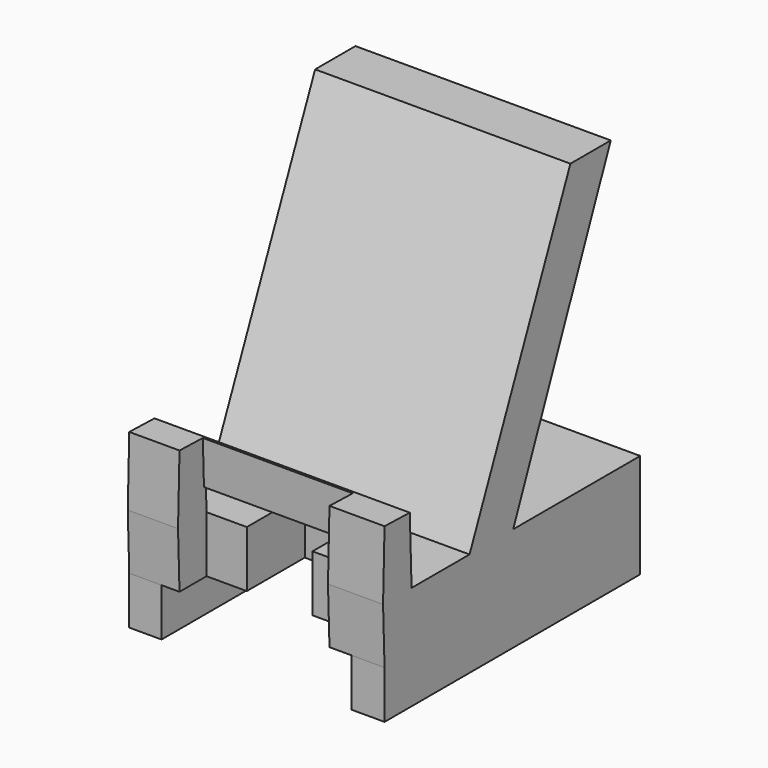
from build123d import *

# Parameters (mm, degrees)
F1_DEPTH  = 80
F2_W      = 10.1163312793
F2_H      = 100.1585014164
F2_W_2    = 10.3900524974
F3_DEPTH  = 15
F6_W      = 19.9106484652
F6_H      = 22.7042857278
F7_DEPTH  = 17.6
F8_W      = 20.5874107778
F8_H      = 22.7042857278
F9_DEPTH  = 17.7
F10_W     = 46.9934158027
F10_H     = 17.6760927897
F10_H_2   = 21.9856097649
F11_DEPTH = 10.4
F13_DEPTH = 25
F15_DEPTH = 25


# Not quite as in the source:
# - a feature of the source that left no trace in its solid (it failed there, or was rolled back) is left out


with BuildPart() as f1:
    # F0 (on Right) → F1 (new body)
    with BuildSketch(Plane.YZ):
        Polygon((22.4307589233, 109.4066873193), (-17.082426697, 17.6664423198), (0, 17.6664423198), (38.2366999984, 109.4066873193), align=None)
        Polygon((-39.7867124248, 17.6664423198), (-39.2026986647, 0), (49.7872419655, 0), (49.7872419655, 17.6664423198), (0, 17.6664423198), (-17.082426697, 17.6664423198), align=None)
        Polygon((-50.955273211, 17.6664423198), (-50.3712594509, 0), (-39.2026986647, 0), (-39.7867124248, 17.6664423198), align=None)
        Polygon((-50.3712594509, 38.982976228), (-50.955273211, 17.6664423198), (-39.7867124248, 17.6664423198), (-40.4824339626, 38.7120499047), align=None)
    extrude(amount=F1_DEPTH)

    # F2 (on face) → F3 (join)
    with BuildSketch(Plane(origin=(0, 0, 0), x_dir=(1, 0, 0), z_dir=(0, 0, -1))):
        with Locations((5.0581656396, 0.2920087427)):
            Rectangle(F2_W, F2_H)
        with Locations((74.8049737513, 0.2920087427)):
            Rectangle(F2_W_2, F2_H)
    extrude(amount=F3_DEPTH)

    # F6 (on face) → F7 (join)
    with BuildSketch(Plane.XY.offset(17.6664423198)):
        with Locations((39.5665168762, -28.4345695609)):
            Rectangle(F6_W, F6_H)
    extrude(amount=-F7_DEPTH)

    # F8 (on face) → F9 (cut)
    with BuildSketch(Plane.XY.offset(17.6664423198)):
        with Locations((38.6653598398, -28.4345695609)):
            Rectangle(F8_W, F8_H)
    extrude(amount=-F9_DEPTH, mode=Mode.SUBTRACT)

    # F10 (on face) → F11 (cut)
    with BuildSketch(Plane(origin=(0, -50.316272907, -1.6633454095), x_dir=(1, 0, 0), z_dir=(0, -0.9994540383, -0.0330397541))):
        with Locations((39.2467323691, 10.5023004233)):
            Rectangle(F10_W, F10_H)
        with Locations((39.2467323691, 30.3331517006)):
            Rectangle(F10_W, F10_H_2)
    extrude(amount=-F11_DEPTH, mode=Mode.SUBTRACT)

    # F12 (on face) → F13 (cut)
    with BuildSketch(Plane(origin=(0, 0, 0), x_dir=(1, 0, 0), z_dir=(0, 0, -1))):
        Polygon((62.7434402704, 50.3712594509), (15.7500244677, 50.3712594509), (15.7500244677, 40.7608151436), (65.7564029098, 40.7608151436), (65.7564029098, 50.3712594509), align=None)
    extrude(amount=-F13_DEPTH, mode=Mode.SUBTRACT)

    # F14 (on face) → F15 (cut)
    with BuildSketch(Plane(origin=(0, 0, 0), x_dir=(1, 0, 0), z_dir=(0, 0, -1))):
        Polygon((62.1888265014, 40.7608151436), (15.7500244677, 40.7608151436), (15.7500244677, 39.7867124248), (28.3716544509, 39.7867124248), (48.9590652287, 39.7867124248), (62.1888265014, 39.7867124248), align=None)
    extrude(amount=-F15_DEPTH, mode=Mode.SUBTRACT)


solid = f1.part
